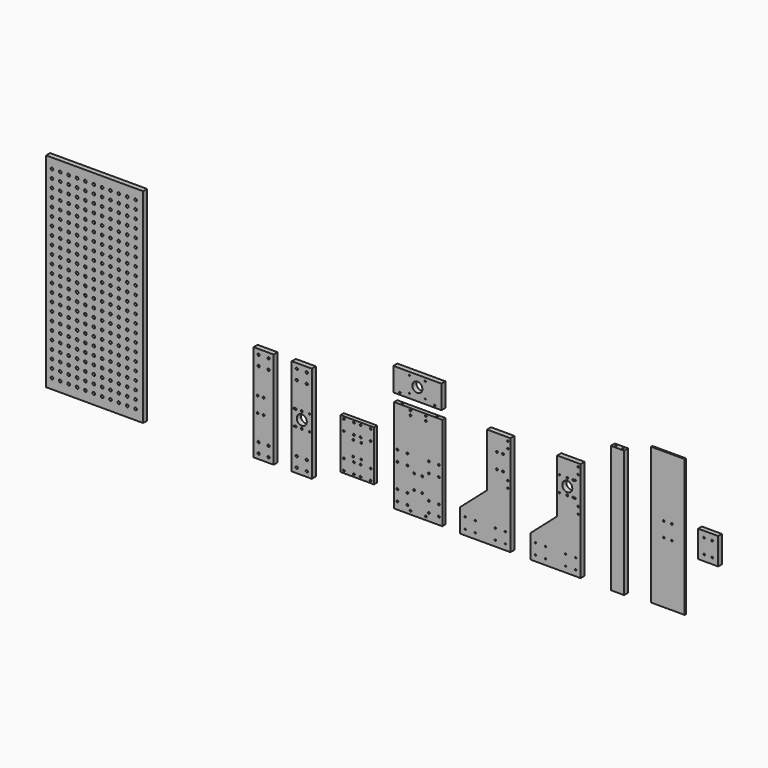
from build123d import *

# Parameters (mm, degrees)
F0_W     = 40
F0_H     = 380
F1_DEPTH = 15
F0_R     = 2.1
F0_R_2   = 2.25
F0_R_3   = 2
F0_R_4   = 2.75
F0_R_5   = 15
F0_W_2   = 60
F0_H_2   = 290
F0_R_6   = 3.4
F0_W_3   = 144
F0_H_3   = 70
F0_R_7   = 2.5
F0_R_8   = 1.8209797518
F0_R_9   = 1.6005552441
F0_R_10  = 1.752522135
F0_R_11  = 1.8797549558
F0_W_4   = 290
F0_H_4   = 610
F0_R_12  = 4
F0_W_5   = 100
F0_H_5   = 410
F2_DEPTH = 5
F0_H_6   = 280
F3_DEPTH = 12
F0_H_7   = 150
F0_H_8   = 80
F4_DEPTH = 14
F5_R     = 2.25
F6_DEPTH = 394.7827727966
F7_R     = 2.5
F8_DEPTH = 10


# Not quite as in the source:
# - a feature names something its author has since deleted; it is built from what else it names


with BuildPart() as f1:
    # F0 (on Front) → F1 (new body)
    with BuildSketch(Plane.XZ):
        with Locations((180, 65.6040832443)):
            Rectangle(F0_W, F0_H)
    extrude(amount=F1_DEPTH)

    # F5 (on face) → F6 (cut, through all)
    with BuildSketch(Plane.XY.offset(255.6040832443)):
        with Locations((170, -7.5)):
            Circle(F5_R)
        with Locations((190, -7.5)):
            Circle(F5_R)
    extrude(amount=-F6_DEPTH, mode=Mode.SUBTRACT)


with BuildPart() as f1b:
    # F0 (on Front) → F1, piece 2 (new body)
    with BuildSketch(Plane.XZ):
        Polygon((-80, -52), (-80, -122), (70, -122), (70, 178), (0, 178), (0, 18), align=None)
        with Locations((-65, -105)):
            Circle(F0_R, mode=Mode.SUBTRACT)
        with Locations((-35, -105)):
            Circle(F0_R, mode=Mode.SUBTRACT)
        with Locations((-65, -73)):
            Circle(F0_R, mode=Mode.SUBTRACT)
        with Locations((-35, -73)):
            Circle(F0_R, mode=Mode.SUBTRACT)
        with Locations((25, -105)):
            Circle(F0_R, mode=Mode.SUBTRACT)
        with Locations((55, -105)):
            Circle(F0_R, mode=Mode.SUBTRACT)
        with Locations((25, -73)):
            Circle(F0_R, mode=Mode.SUBTRACT)
        with Locations((55, -73)):
            Circle(F0_R, mode=Mode.SUBTRACT)
        with Locations((62.5, 44)):
            Circle(F0_R_2, mode=Mode.SUBTRACT)
        with Locations((62.5, 64)):
            Circle(F0_R_2, mode=Mode.SUBTRACT)
        with Locations((6.5, 82.5)):
            Circle(F0_R_3, mode=Mode.SUBTRACT)
        with Locations((30, 83)):
            Circle(F0_R_4, mode=Mode.SUBTRACT)
        with Locations((48, 83)):
            Circle(F0_R_4, mode=Mode.SUBTRACT)
        with Locations((53.5, 82.5)):
            Circle(F0_R_3, mode=Mode.SUBTRACT)
        with Locations((30, 106)):
            Circle(F0_R_5, mode=Mode.SUBTRACT)
        with Locations((6.5, 129.5)):
            Circle(F0_R_3, mode=Mode.SUBTRACT)
        with Locations((30, 129)):
            Circle(F0_R_4, mode=Mode.SUBTRACT)
        with Locations((48, 129)):
            Circle(F0_R_4, mode=Mode.SUBTRACT)
        with Locations((53.5, 130.2057206631)):
            Circle(F0_R_3, mode=Mode.SUBTRACT)
        with Locations((62.5, 148)):
            Circle(F0_R_2, mode=Mode.SUBTRACT)
        with Locations((62.5, 168)):
            Circle(F0_R_2, mode=Mode.SUBTRACT)
    extrude(amount=F1_DEPTH)


with BuildPart() as f1c:
    # F0 (on Front) → F1, piece 3 (new body)
    with BuildSketch(Plane.XZ):
        Polygon((-290, -52), (-290, -122), (-140, -122), (-140, 178), (-210, 178), (-210, 18), align=None)
        with Locations((-275, -105)):
            Circle(F0_R, mode=Mode.SUBTRACT)
        with Locations((-275, -73)):
            Circle(F0_R, mode=Mode.SUBTRACT)
        with Locations((-245, -105)):
            Circle(F0_R, mode=Mode.SUBTRACT)
        with Locations((-185, -105)):
            Circle(F0_R, mode=Mode.SUBTRACT)
        with Locations((-155, -105)):
            Circle(F0_R, mode=Mode.SUBTRACT)
        with Locations((-245, -73)):
            Circle(F0_R, mode=Mode.SUBTRACT)
        with Locations((-185, -73)):
            Circle(F0_R, mode=Mode.SUBTRACT)
        with Locations((-155, -73)):
            Circle(F0_R, mode=Mode.SUBTRACT)
        with Locations((-147.5, 44)):
            Circle(F0_R_2, mode=Mode.SUBTRACT)
        with Locations((-147.5, 64)):
            Circle(F0_R_2, mode=Mode.SUBTRACT)
        with Locations((-180, 83)):
            Circle(F0_R_4, mode=Mode.SUBTRACT)
        with Locations((-162, 83)):
            Circle(F0_R_4, mode=Mode.SUBTRACT)
        with Locations((-180, 129)):
            Circle(F0_R_4, mode=Mode.SUBTRACT)
        with Locations((-162, 129)):
            Circle(F0_R_4, mode=Mode.SUBTRACT)
        with Locations((-147.5, 148)):
            Circle(F0_R_2, mode=Mode.SUBTRACT)
        with Locations((-147.5, 168)):
            Circle(F0_R_2, mode=Mode.SUBTRACT)
    extrude(amount=F1_DEPTH)


with BuildPart() as f1d:
    # F0 (on Front) → F1, piece 4 (new body)
    with BuildSketch(Plane.XZ):
        with Locations((-763.4110760689, 23)):
            Rectangle(F0_W_2, F0_H_2)
        with Locations((-778.4110760689, -107)):
            Circle(F0_R_6, mode=Mode.SUBTRACT)
        with Locations((-778.4110760689, -77)):
            Circle(F0_R_6, mode=Mode.SUBTRACT)
        with Locations((-748.4110760689, -107)):
            Circle(F0_R_6, mode=Mode.SUBTRACT)
        with Locations((-748.4110760689, -77)):
            Circle(F0_R_6, mode=Mode.SUBTRACT)
        with Locations((-786.9110760689, -0.5)):
            Circle(F0_R_3, mode=Mode.SUBTRACT)
        with Locations((-781.4110760689, 0)):
            Circle(F0_R_4, mode=Mode.SUBTRACT)
        with Locations((-763.4110760689, 0)):
            Circle(F0_R_4, mode=Mode.SUBTRACT)
        with Locations((-739.9110760689, -0.5)):
            Circle(F0_R_3, mode=Mode.SUBTRACT)
        with Locations((-786.9110760689, 46.5)):
            Circle(F0_R_3, mode=Mode.SUBTRACT)
        with Locations((-781.4110760689, 46)):
            Circle(F0_R_4, mode=Mode.SUBTRACT)
        with Locations((-763.4110760689, 23)):
            Circle(F0_R_5, mode=Mode.SUBTRACT)
        with Locations((-763.4110760689, 46)):
            Circle(F0_R_4, mode=Mode.SUBTRACT)
        with Locations((-739.9110760689, 46.5)):
            Circle(F0_R_3, mode=Mode.SUBTRACT)
        with Locations((-778.4110760689, 123)):
            Circle(F0_R_6, mode=Mode.SUBTRACT)
        with Locations((-778.4110760689, 153)):
            Circle(F0_R_6, mode=Mode.SUBTRACT)
        with Locations((-748.4110760689, 123)):
            Circle(F0_R_6, mode=Mode.SUBTRACT)
        with Locations((-748.4110760689, 153)):
            Circle(F0_R_6, mode=Mode.SUBTRACT)
    extrude(amount=F1_DEPTH)


with BuildPart() as f1e:
    # F0 (on Front) → F1, piece 5 (new body)
    with BuildSketch(Plane.XZ):
        with Locations((-877.410800457, 23)):
            Rectangle(F0_W_2, F0_H_2)
        with Locations((-892.410800457, -107)):
            Circle(F0_R_6, mode=Mode.SUBTRACT)
        with Locations((-862.410800457, -107)):
            Circle(F0_R_6, mode=Mode.SUBTRACT)
        with Locations((-892.410800457, -77)):
            Circle(F0_R_6, mode=Mode.SUBTRACT)
        with Locations((-862.410800457, -77)):
            Circle(F0_R_6, mode=Mode.SUBTRACT)
        with Locations((-895.410800457, -1.2824487388)):
            Circle(F0_R_4, mode=Mode.SUBTRACT)
        with Locations((-877.410800457, -1.2824487388)):
            Circle(F0_R_4, mode=Mode.SUBTRACT)
        with Locations((-895.410800457, 44.7175512612)):
            Circle(F0_R_4, mode=Mode.SUBTRACT)
        with Locations((-877.410800457, 44.7175512612)):
            Circle(F0_R_4, mode=Mode.SUBTRACT)
        with Locations((-892.410800457, 123)):
            Circle(F0_R_6, mode=Mode.SUBTRACT)
        with Locations((-862.410800457, 123)):
            Circle(F0_R_6, mode=Mode.SUBTRACT)
        with Locations((-892.410800457, 153)):
            Circle(F0_R_6, mode=Mode.SUBTRACT)
        with Locations((-862.410800457, 153)):
            Circle(F0_R_6, mode=Mode.SUBTRACT)
    extrude(amount=F1_DEPTH)


with BuildPart() as f1f:
    # F0 (on Front) → F1, piece 6 (new body)
    with BuildSketch(Plane.XZ):
        with Locations((-418, 219.5401751995)):
            Rectangle(F0_W_3, F0_H_3)
        with Locations((-470, 190.5401751995)):
            Circle(F0_R_7, mode=Mode.SUBTRACT)
        with Locations((-441.5, 198.0401751995)):
            Circle(F0_R_8, mode=Mode.SUBTRACT)
        with Locations((-366, 190.5401751995)):
            Circle(F0_R_7, mode=Mode.SUBTRACT)
        with Locations((-394.5, 198.0401751995)):
            Circle(F0_R_9, mode=Mode.SUBTRACT)
        with Locations((-418, 221.5401751995)):
            Circle(F0_R_5, mode=Mode.SUBTRACT)
        with Locations((-441.5, 245.0401751995)):
            Circle(F0_R_10, mode=Mode.SUBTRACT)
        with Locations((-394.5, 245.0401751995)):
            Circle(F0_R_11, mode=Mode.SUBTRACT)
    extrude(amount=F1_DEPTH)


with BuildPart() as f1g:
    # F0 (on Front) → F1, piece 7 (new body)
    with BuildSketch(Plane.XZ):
        with Locations((-1382.5847482681, 165.8223104477)):
            Rectangle(F0_W_4, F0_H_4)
        with Locations((-1510.0847482681, -109.1776895523)):
            Circle(F0_R_12, mode=Mode.SUBTRACT)
        with Locations((-1485.0847482681, -109.1776895523)):
            Circle(F0_R_12, mode=Mode.SUBTRACT)
        with Locations((-1460.0847482681, -109.1776895523)):
            Circle(F0_R_12, mode=Mode.SUBTRACT)
        with Locations((-1435.0847482681, -109.1776895523)):
            Circle(F0_R_12, mode=Mode.SUBTRACT)
        with Locations((-1410.0847482681, -109.1776895523)):
            Circle(F0_R_12, mode=Mode.SUBTRACT)
        with Locations((-1385.0847482681, -109.1776895523)):
            Circle(F0_R_12, mode=Mode.SUBTRACT)
        with Locations((-1360.0847482681, -109.1776895523)):
            Circle(F0_R_12, mode=Mode.SUBTRACT)
        with Locations((-1335.0847482681, -109.1776895523)):
            Circle(F0_R_12, mode=Mode.SUBTRACT)
        with Locations((-1310.0847482681, -109.1776895523)):
            Circle(F0_R_12, mode=Mode.SUBTRACT)
        with Locations((-1285.0847482681, -109.1776895523)):
            Circle(F0_R_12, mode=Mode.SUBTRACT)
        with Locations((-1510.0847482681, -84.1776895523)):
            Circle(F0_R_12, mode=Mode.SUBTRACT)
        with Locations((-1485.0847482681, -84.1776895523)):
            Circle(F0_R_12, mode=Mode.SUBTRACT)
        with Locations((-1460.0847482681, -84.1776895523)):
            Circle(F0_R_12, mode=Mode.SUBTRACT)
        with Locations((-1435.0847482681, -84.1776895523)):
            Circle(F0_R_12, mode=Mode.SUBTRACT)
        with Locations((-1410.0847482681, -84.1776895523)):
            Circle(F0_R_12, mode=Mode.SUBTRACT)
        with Locations((-1385.0847482681, -84.1776895523)):
            Circle(F0_R_12, mode=Mode.SUBTRACT)
        with Locations((-1360.0847482681, -84.1776895523)):
            Circle(F0_R_12, mode=Mode.SUBTRACT)
        with Locations((-1335.0847482681, -84.1776895523)):
            Circle(F0_R_12, mode=Mode.SUBTRACT)
        with Locations((-1310.0847482681, -84.1776895523)):
            Circle(F0_R_12, mode=Mode.SUBTRACT)
        with Locations((-1285.0847482681, -84.1776895523)):
            Circle(F0_R_12, mode=Mode.SUBTRACT)
        with Locations((-1260.0847482681, -109.1776895523)):
            Circle(F0_R_12, mode=Mode.SUBTRACT)
        with Locations((-1260.0847482681, -84.1776895523)):
            Circle(F0_R_12, mode=Mode.SUBTRACT)
        with Locations((-1510.0847482681, -59.1776895523)):
            Circle(F0_R_12, mode=Mode.SUBTRACT)
        with Locations((-1485.0847482681, -59.1776895523)):
            Circle(F0_R_12, mode=Mode.SUBTRACT)
        with Locations((-1460.0847482681, -59.1776895523)):
            Circle(F0_R_12, mode=Mode.SUBTRACT)
        with Locations((-1435.0847482681, -59.1776895523)):
            Circle(F0_R_12, mode=Mode.SUBTRACT)
        with Locations((-1410.0847482681, -59.1776895523)):
            Circle(F0_R_12, mode=Mode.SUBTRACT)
        with Locations((-1510.0847482681, -34.1776895523)):
            Circle(F0_R_12, mode=Mode.SUBTRACT)
        with Locations((-1485.0847482681, -34.1776895523)):
            Circle(F0_R_12, mode=Mode.SUBTRACT)
        with Locations((-1460.0847482681, -34.1776895523)):
            Circle(F0_R_12, mode=Mode.SUBTRACT)
        with Locations((-1435.0847482681, -34.1776895523)):
            Circle(F0_R_12, mode=Mode.SUBTRACT)
        with Locations((-1410.0847482681, -34.1776895523)):
            Circle(F0_R_12, mode=Mode.SUBTRACT)
        with Locations((-1385.0847482681, -59.1776895523)):
            Circle(F0_R_12, mode=Mode.SUBTRACT)
        with Locations((-1360.0847482681, -59.1776895523)):
            Circle(F0_R_12, mode=Mode.SUBTRACT)
        with Locations((-1335.0847482681, -59.1776895523)):
            Circle(F0_R_12, mode=Mode.SUBTRACT)
        with Locations((-1310.0847482681, -59.1776895523)):
            Circle(F0_R_12, mode=Mode.SUBTRACT)
        with Locations((-1285.0847482681, -59.1776895523)):
            Circle(F0_R_12, mode=Mode.SUBTRACT)
        with Locations((-1385.0847482681, -34.1776895523)):
            Circle(F0_R_12, mode=Mode.SUBTRACT)
        with Locations((-1360.0847482681, -34.1776895523)):
            Circle(F0_R_12, mode=Mode.SUBTRACT)
        with Locations((-1335.0847482681, -34.1776895523)):
            Circle(F0_R_12, mode=Mode.SUBTRACT)
        with Locations((-1310.0847482681, -34.1776895523)):
            Circle(F0_R_12, mode=Mode.SUBTRACT)
        with Locations((-1285.0847482681, -34.1776895523)):
            Circle(F0_R_12, mode=Mode.SUBTRACT)
        with Locations((-1510.0847482681, -9.1776895523)):
            Circle(F0_R_12, mode=Mode.SUBTRACT)
        with Locations((-1485.0847482681, -9.1776895523)):
            Circle(F0_R_12, mode=Mode.SUBTRACT)
        with Locations((-1460.0847482681, -9.1776895523)):
            Circle(F0_R_12, mode=Mode.SUBTRACT)
        with Locations((-1435.0847482681, -9.1776895523)):
            Circle(F0_R_12, mode=Mode.SUBTRACT)
        with Locations((-1410.0847482681, -9.1776895523)):
            Circle(F0_R_12, mode=Mode.SUBTRACT)
        with Locations((-1385.0847482681, -9.1776895523)):
            Circle(F0_R_12, mode=Mode.SUBTRACT)
        with Locations((-1360.0847482681, -9.1776895523)):
            Circle(F0_R_12, mode=Mode.SUBTRACT)
        with Locations((-1335.0847482681, -9.1776895523)):
            Circle(F0_R_12, mode=Mode.SUBTRACT)
        with Locations((-1310.0847482681, -9.1776895523)):
            Circle(F0_R_12, mode=Mode.SUBTRACT)
        with Locations((-1285.0847482681, -9.1776895523)):
            Circle(F0_R_12, mode=Mode.SUBTRACT)
        with Locations((-1260.0847482681, -59.1776895523)):
            Circle(F0_R_12, mode=Mode.SUBTRACT)
        with Locations((-1260.0847482681, -34.1776895523)):
            Circle(F0_R_12, mode=Mode.SUBTRACT)
        with Locations((-1260.0847482681, -9.1776895523)):
            Circle(F0_R_12, mode=Mode.SUBTRACT)
        with Locations((-1510.0847482681, 15.8223104477)):
            Circle(F0_R_12, mode=Mode.SUBTRACT)
        with Locations((-1485.0847482681, 15.8223104477)):
            Circle(F0_R_12, mode=Mode.SUBTRACT)
        with Locations((-1460.0847482681, 15.8223104477)):
            Circle(F0_R_12, mode=Mode.SUBTRACT)
        with Locations((-1435.0847482681, 15.8223104477)):
            Circle(F0_R_12, mode=Mode.SUBTRACT)
        with Locations((-1410.0847482681, 15.8223104477)):
            Circle(F0_R_12, mode=Mode.SUBTRACT)
        with Locations((-1510.0847482681, 40.8223104477)):
            Circle(F0_R_12, mode=Mode.SUBTRACT)
        with Locations((-1485.0847482681, 40.8223104477)):
            Circle(F0_R_12, mode=Mode.SUBTRACT)
        with Locations((-1460.0847482681, 40.8223104477)):
            Circle(F0_R_12, mode=Mode.SUBTRACT)
        with Locations((-1435.0847482681, 40.8223104477)):
            Circle(F0_R_12, mode=Mode.SUBTRACT)
        with Locations((-1410.0847482681, 40.8223104477)):
            Circle(F0_R_12, mode=Mode.SUBTRACT)
        with Locations((-1385.0847482681, 15.8223104477)):
            Circle(F0_R_12, mode=Mode.SUBTRACT)
        with Locations((-1360.0847482681, 15.8223104477)):
            Circle(F0_R_12, mode=Mode.SUBTRACT)
        with Locations((-1335.0847482681, 15.8223104477)):
            Circle(F0_R_12, mode=Mode.SUBTRACT)
        with Locations((-1310.0847482681, 15.8223104477)):
            Circle(F0_R_12, mode=Mode.SUBTRACT)
        with Locations((-1285.0847482681, 15.8223104477)):
            Circle(F0_R_12, mode=Mode.SUBTRACT)
        with Locations((-1385.0847482681, 40.8223104477)):
            Circle(F0_R_12, mode=Mode.SUBTRACT)
        with Locations((-1360.0847482681, 40.8223104477)):
            Circle(F0_R_12, mode=Mode.SUBTRACT)
        with Locations((-1335.0847482681, 40.8223104477)):
            Circle(F0_R_12, mode=Mode.SUBTRACT)
        with Locations((-1310.0847482681, 40.8223104477)):
            Circle(F0_R_12, mode=Mode.SUBTRACT)
        with Locations((-1285.0847482681, 40.8223104477)):
            Circle(F0_R_12, mode=Mode.SUBTRACT)
        with Locations((-1510.0847482681, 65.8223104477)):
            Circle(F0_R_12, mode=Mode.SUBTRACT)
        with Locations((-1485.0847482681, 65.8223104477)):
            Circle(F0_R_12, mode=Mode.SUBTRACT)
        with Locations((-1460.0847482681, 65.8223104477)):
            Circle(F0_R_12, mode=Mode.SUBTRACT)
        with Locations((-1435.0847482681, 65.8223104477)):
            Circle(F0_R_12, mode=Mode.SUBTRACT)
        with Locations((-1410.0847482681, 65.8223104477)):
            Circle(F0_R_12, mode=Mode.SUBTRACT)
        with Locations((-1385.0847482681, 65.8223104477)):
            Circle(F0_R_12, mode=Mode.SUBTRACT)
        with Locations((-1360.0847482681, 65.8223104477)):
            Circle(F0_R_12, mode=Mode.SUBTRACT)
        with Locations((-1335.0847482681, 65.8223104477)):
            Circle(F0_R_12, mode=Mode.SUBTRACT)
        with Locations((-1310.0847482681, 65.8223104477)):
            Circle(F0_R_12, mode=Mode.SUBTRACT)
        with Locations((-1285.0847482681, 65.8223104477)):
            Circle(F0_R_12, mode=Mode.SUBTRACT)
        with Locations((-1260.0847482681, 15.8223104477)):
            Circle(F0_R_12, mode=Mode.SUBTRACT)
        with Locations((-1260.0847482681, 40.8223104477)):
            Circle(F0_R_12, mode=Mode.SUBTRACT)
        with Locations((-1260.0847482681, 65.8223104477)):
            Circle(F0_R_12, mode=Mode.SUBTRACT)
        with Locations((-1510.0847482681, 90.8223104477)):
            Circle(F0_R_12, mode=Mode.SUBTRACT)
        with Locations((-1485.0847482681, 90.8223104477)):
            Circle(F0_R_12, mode=Mode.SUBTRACT)
        with Locations((-1460.0847482681, 90.8223104477)):
            Circle(F0_R_12, mode=Mode.SUBTRACT)
        with Locations((-1435.0847482681, 90.8223104477)):
            Circle(F0_R_12, mode=Mode.SUBTRACT)
        with Locations((-1410.0847482681, 90.8223104477)):
            Circle(F0_R_12, mode=Mode.SUBTRACT)
        with Locations((-1510.0847482681, 115.8223104477)):
            Circle(F0_R_12, mode=Mode.SUBTRACT)
        with Locations((-1485.0847482681, 115.8223104477)):
            Circle(F0_R_12, mode=Mode.SUBTRACT)
        with Locations((-1460.0847482681, 115.8223104477)):
            Circle(F0_R_12, mode=Mode.SUBTRACT)
        with Locations((-1435.0847482681, 115.8223104477)):
            Circle(F0_R_12, mode=Mode.SUBTRACT)
        with Locations((-1410.0847482681, 115.8223104477)):
            Circle(F0_R_12, mode=Mode.SUBTRACT)
        with Locations((-1385.0847482681, 90.8223104477)):
            Circle(F0_R_12, mode=Mode.SUBTRACT)
        with Locations((-1360.0847482681, 90.8223104477)):
            Circle(F0_R_12, mode=Mode.SUBTRACT)
        with Locations((-1335.0847482681, 90.8223104477)):
            Circle(F0_R_12, mode=Mode.SUBTRACT)
        with Locations((-1310.0847482681, 90.8223104477)):
            Circle(F0_R_12, mode=Mode.SUBTRACT)
        with Locations((-1285.0847482681, 90.8223104477)):
            Circle(F0_R_12, mode=Mode.SUBTRACT)
        with Locations((-1385.0847482681, 115.8223104477)):
            Circle(F0_R_12, mode=Mode.SUBTRACT)
        with Locations((-1360.0847482681, 115.8223104477)):
            Circle(F0_R_12, mode=Mode.SUBTRACT)
        with Locations((-1335.0847482681, 115.8223104477)):
            Circle(F0_R_12, mode=Mode.SUBTRACT)
        with Locations((-1310.0847482681, 115.8223104477)):
            Circle(F0_R_12, mode=Mode.SUBTRACT)
        with Locations((-1285.0847482681, 115.8223104477)):
            Circle(F0_R_12, mode=Mode.SUBTRACT)
        with Locations((-1510.0847482681, 140.8223104477)):
            Circle(F0_R_12, mode=Mode.SUBTRACT)
        with Locations((-1485.0847482681, 140.8223104477)):
            Circle(F0_R_12, mode=Mode.SUBTRACT)
        with Locations((-1460.0847482681, 140.8223104477)):
            Circle(F0_R_12, mode=Mode.SUBTRACT)
        with Locations((-1435.0847482681, 140.8223104477)):
            Circle(F0_R_12, mode=Mode.SUBTRACT)
        with Locations((-1410.0847482681, 140.8223104477)):
            Circle(F0_R_12, mode=Mode.SUBTRACT)
        with Locations((-1385.0847482681, 140.8223104477)):
            Circle(F0_R_12, mode=Mode.SUBTRACT)
        with Locations((-1360.0847482681, 140.8223104477)):
            Circle(F0_R_12, mode=Mode.SUBTRACT)
        with Locations((-1335.0847482681, 140.8223104477)):
            Circle(F0_R_12, mode=Mode.SUBTRACT)
        with Locations((-1310.0847482681, 140.8223104477)):
            Circle(F0_R_12, mode=Mode.SUBTRACT)
        with Locations((-1285.0847482681, 140.8223104477)):
            Circle(F0_R_12, mode=Mode.SUBTRACT)
        with Locations((-1260.0847482681, 90.8223104477)):
            Circle(F0_R_12, mode=Mode.SUBTRACT)
        with Locations((-1260.0847482681, 115.8223104477)):
            Circle(F0_R_12, mode=Mode.SUBTRACT)
        with Locations((-1260.0847482681, 140.8223104477)):
            Circle(F0_R_12, mode=Mode.SUBTRACT)
        with Locations((-1510.0847482681, 165.8223104477)):
            Circle(F0_R_12, mode=Mode.SUBTRACT)
        with Locations((-1485.0847482681, 165.8223104477)):
            Circle(F0_R_12, mode=Mode.SUBTRACT)
        with Locations((-1460.0847482681, 165.8223104477)):
            Circle(F0_R_12, mode=Mode.SUBTRACT)
        with Locations((-1435.0847482681, 165.8223104477)):
            Circle(F0_R_12, mode=Mode.SUBTRACT)
        with Locations((-1410.0847482681, 165.8223104477)):
            Circle(F0_R_12, mode=Mode.SUBTRACT)
        with Locations((-1510.0847482681, 190.8223104477)):
            Circle(F0_R_12, mode=Mode.SUBTRACT)
        with Locations((-1485.0847482681, 190.8223104477)):
            Circle(F0_R_12, mode=Mode.SUBTRACT)
        with Locations((-1460.0847482681, 190.8223104477)):
            Circle(F0_R_12, mode=Mode.SUBTRACT)
        with Locations((-1435.0847482681, 190.8223104477)):
            Circle(F0_R_12, mode=Mode.SUBTRACT)
        with Locations((-1410.0847482681, 190.8223104477)):
            Circle(F0_R_12, mode=Mode.SUBTRACT)
        with Locations((-1385.0847482681, 165.8223104477)):
            Circle(F0_R_12, mode=Mode.SUBTRACT)
        with Locations((-1360.0847482681, 165.8223104477)):
            Circle(F0_R_12, mode=Mode.SUBTRACT)
        with Locations((-1335.0847482681, 165.8223104477)):
            Circle(F0_R_12, mode=Mode.SUBTRACT)
        with Locations((-1310.0847482681, 165.8223104477)):
            Circle(F0_R_12, mode=Mode.SUBTRACT)
        with Locations((-1285.0847482681, 165.8223104477)):
            Circle(F0_R_12, mode=Mode.SUBTRACT)
        with Locations((-1385.0847482681, 190.8223104477)):
            Circle(F0_R_12, mode=Mode.SUBTRACT)
        with Locations((-1360.0847482681, 190.8223104477)):
            Circle(F0_R_12, mode=Mode.SUBTRACT)
        with Locations((-1335.0847482681, 190.8223104477)):
            Circle(F0_R_12, mode=Mode.SUBTRACT)
        with Locations((-1310.0847482681, 190.8223104477)):
            Circle(F0_R_12, mode=Mode.SUBTRACT)
        with Locations((-1285.0847482681, 190.8223104477)):
            Circle(F0_R_12, mode=Mode.SUBTRACT)
        with Locations((-1510.0847482681, 215.8223104477)):
            Circle(F0_R_12, mode=Mode.SUBTRACT)
        with Locations((-1485.0847482681, 215.8223104477)):
            Circle(F0_R_12, mode=Mode.SUBTRACT)
        with Locations((-1460.0847482681, 215.8223104477)):
            Circle(F0_R_12, mode=Mode.SUBTRACT)
        with Locations((-1435.0847482681, 215.8223104477)):
            Circle(F0_R_12, mode=Mode.SUBTRACT)
        with Locations((-1410.0847482681, 215.8223104477)):
            Circle(F0_R_12, mode=Mode.SUBTRACT)
        with Locations((-1510.0847482681, 240.8223104477)):
            Circle(F0_R_12, mode=Mode.SUBTRACT)
        with Locations((-1485.0847482681, 240.8223104477)):
            Circle(F0_R_12, mode=Mode.SUBTRACT)
        with Locations((-1460.0847482681, 240.8223104477)):
            Circle(F0_R_12, mode=Mode.SUBTRACT)
        with Locations((-1435.0847482681, 240.8223104477)):
            Circle(F0_R_12, mode=Mode.SUBTRACT)
        with Locations((-1410.0847482681, 240.8223104477)):
            Circle(F0_R_12, mode=Mode.SUBTRACT)
        with Locations((-1385.0847482681, 215.8223104477)):
            Circle(F0_R_12, mode=Mode.SUBTRACT)
        with Locations((-1360.0847482681, 215.8223104477)):
            Circle(F0_R_12, mode=Mode.SUBTRACT)
        with Locations((-1335.0847482681, 215.8223104477)):
            Circle(F0_R_12, mode=Mode.SUBTRACT)
        with Locations((-1310.0847482681, 215.8223104477)):
            Circle(F0_R_12, mode=Mode.SUBTRACT)
        with Locations((-1285.0847482681, 215.8223104477)):
            Circle(F0_R_12, mode=Mode.SUBTRACT)
        with Locations((-1385.0847482681, 240.8223104477)):
            Circle(F0_R_12, mode=Mode.SUBTRACT)
        with Locations((-1360.0847482681, 240.8223104477)):
            Circle(F0_R_12, mode=Mode.SUBTRACT)
        with Locations((-1335.0847482681, 240.8223104477)):
            Circle(F0_R_12, mode=Mode.SUBTRACT)
        with Locations((-1310.0847482681, 240.8223104477)):
            Circle(F0_R_12, mode=Mode.SUBTRACT)
        with Locations((-1285.0847482681, 240.8223104477)):
            Circle(F0_R_12, mode=Mode.SUBTRACT)
        with Locations((-1260.0847482681, 165.8223104477)):
            Circle(F0_R_12, mode=Mode.SUBTRACT)
        with Locations((-1260.0847482681, 190.8223104477)):
            Circle(F0_R_12, mode=Mode.SUBTRACT)
        with Locations((-1260.0847482681, 215.8223104477)):
            Circle(F0_R_12, mode=Mode.SUBTRACT)
        with Locations((-1260.0847482681, 240.8223104477)):
            Circle(F0_R_12, mode=Mode.SUBTRACT)
        with Locations((-1510.0847482681, 265.8223104477)):
            Circle(F0_R_12, mode=Mode.SUBTRACT)
        with Locations((-1485.0847482681, 265.8223104477)):
            Circle(F0_R_12, mode=Mode.SUBTRACT)
        with Locations((-1460.0847482681, 265.8223104477)):
            Circle(F0_R_12, mode=Mode.SUBTRACT)
        with Locations((-1435.0847482681, 265.8223104477)):
            Circle(F0_R_12, mode=Mode.SUBTRACT)
        with Locations((-1410.0847482681, 265.8223104477)):
            Circle(F0_R_12, mode=Mode.SUBTRACT)
        with Locations((-1385.0847482681, 265.8223104477)):
            Circle(F0_R_12, mode=Mode.SUBTRACT)
        with Locations((-1360.0847482681, 265.8223104477)):
            Circle(F0_R_12, mode=Mode.SUBTRACT)
        with Locations((-1335.0847482681, 265.8223104477)):
            Circle(F0_R_12, mode=Mode.SUBTRACT)
        with Locations((-1310.0847482681, 265.8223104477)):
            Circle(F0_R_12, mode=Mode.SUBTRACT)
        with Locations((-1285.0847482681, 265.8223104477)):
            Circle(F0_R_12, mode=Mode.SUBTRACT)
        with Locations((-1510.0847482681, 290.8223104477)):
            Circle(F0_R_12, mode=Mode.SUBTRACT)
        with Locations((-1485.0847482681, 290.8223104477)):
            Circle(F0_R_12, mode=Mode.SUBTRACT)
        with Locations((-1460.0847482681, 290.8223104477)):
            Circle(F0_R_12, mode=Mode.SUBTRACT)
        with Locations((-1435.0847482681, 290.8223104477)):
            Circle(F0_R_12, mode=Mode.SUBTRACT)
        with Locations((-1410.0847482681, 290.8223104477)):
            Circle(F0_R_12, mode=Mode.SUBTRACT)
        with Locations((-1510.0847482681, 315.8223104477)):
            Circle(F0_R_12, mode=Mode.SUBTRACT)
        with Locations((-1485.0847482681, 315.8223104477)):
            Circle(F0_R_12, mode=Mode.SUBTRACT)
        with Locations((-1460.0847482681, 315.8223104477)):
            Circle(F0_R_12, mode=Mode.SUBTRACT)
        with Locations((-1435.0847482681, 315.8223104477)):
            Circle(F0_R_12, mode=Mode.SUBTRACT)
        with Locations((-1410.0847482681, 315.8223104477)):
            Circle(F0_R_12, mode=Mode.SUBTRACT)
        with Locations((-1385.0847482681, 290.8223104477)):
            Circle(F0_R_12, mode=Mode.SUBTRACT)
        with Locations((-1360.0847482681, 290.8223104477)):
            Circle(F0_R_12, mode=Mode.SUBTRACT)
        with Locations((-1335.0847482681, 290.8223104477)):
            Circle(F0_R_12, mode=Mode.SUBTRACT)
        with Locations((-1310.0847482681, 290.8223104477)):
            Circle(F0_R_12, mode=Mode.SUBTRACT)
        with Locations((-1285.0847482681, 290.8223104477)):
            Circle(F0_R_12, mode=Mode.SUBTRACT)
        with Locations((-1385.0847482681, 315.8223104477)):
            Circle(F0_R_12, mode=Mode.SUBTRACT)
        with Locations((-1360.0847482681, 315.8223104477)):
            Circle(F0_R_12, mode=Mode.SUBTRACT)
        with Locations((-1335.0847482681, 315.8223104477)):
            Circle(F0_R_12, mode=Mode.SUBTRACT)
        with Locations((-1310.0847482681, 315.8223104477)):
            Circle(F0_R_12, mode=Mode.SUBTRACT)
        with Locations((-1285.0847482681, 315.8223104477)):
            Circle(F0_R_12, mode=Mode.SUBTRACT)
        with Locations((-1260.0847482681, 265.8223104477)):
            Circle(F0_R_12, mode=Mode.SUBTRACT)
        with Locations((-1260.0847482681, 290.8223104477)):
            Circle(F0_R_12, mode=Mode.SUBTRACT)
        with Locations((-1260.0847482681, 315.8223104477)):
            Circle(F0_R_12, mode=Mode.SUBTRACT)
        with Locations((-1510.0847482681, 340.8223104477)):
            Circle(F0_R_12, mode=Mode.SUBTRACT)
        with Locations((-1485.0847482681, 340.8223104477)):
            Circle(F0_R_12, mode=Mode.SUBTRACT)
        with Locations((-1460.0847482681, 340.8223104477)):
            Circle(F0_R_12, mode=Mode.SUBTRACT)
        with Locations((-1435.0847482681, 340.8223104477)):
            Circle(F0_R_12, mode=Mode.SUBTRACT)
        with Locations((-1410.0847482681, 340.8223104477)):
            Circle(F0_R_12, mode=Mode.SUBTRACT)
        with Locations((-1385.0847482681, 340.8223104477)):
            Circle(F0_R_12, mode=Mode.SUBTRACT)
        with Locations((-1360.0847482681, 340.8223104477)):
            Circle(F0_R_12, mode=Mode.SUBTRACT)
        with Locations((-1335.0847482681, 340.8223104477)):
            Circle(F0_R_12, mode=Mode.SUBTRACT)
        with Locations((-1310.0847482681, 340.8223104477)):
            Circle(F0_R_12, mode=Mode.SUBTRACT)
        with Locations((-1285.0847482681, 340.8223104477)):
            Circle(F0_R_12, mode=Mode.SUBTRACT)
        with Locations((-1510.0847482681, 365.8223104477)):
            Circle(F0_R_12, mode=Mode.SUBTRACT)
        with Locations((-1485.0847482681, 365.8223104477)):
            Circle(F0_R_12, mode=Mode.SUBTRACT)
        with Locations((-1460.0847482681, 365.8223104477)):
            Circle(F0_R_12, mode=Mode.SUBTRACT)
        with Locations((-1435.0847482681, 365.8223104477)):
            Circle(F0_R_12, mode=Mode.SUBTRACT)
        with Locations((-1410.0847482681, 365.8223104477)):
            Circle(F0_R_12, mode=Mode.SUBTRACT)
        with Locations((-1510.0847482681, 390.8223104477)):
            Circle(F0_R_12, mode=Mode.SUBTRACT)
        with Locations((-1485.0847482681, 390.8223104477)):
            Circle(F0_R_12, mode=Mode.SUBTRACT)
        with Locations((-1460.0847482681, 390.8223104477)):
            Circle(F0_R_12, mode=Mode.SUBTRACT)
        with Locations((-1435.0847482681, 390.8223104477)):
            Circle(F0_R_12, mode=Mode.SUBTRACT)
        with Locations((-1410.0847482681, 390.8223104477)):
            Circle(F0_R_12, mode=Mode.SUBTRACT)
        with Locations((-1385.0847482681, 365.8223104477)):
            Circle(F0_R_12, mode=Mode.SUBTRACT)
        with Locations((-1360.0847482681, 365.8223104477)):
            Circle(F0_R_12, mode=Mode.SUBTRACT)
        with Locations((-1335.0847482681, 365.8223104477)):
            Circle(F0_R_12, mode=Mode.SUBTRACT)
        with Locations((-1310.0847482681, 365.8223104477)):
            Circle(F0_R_12, mode=Mode.SUBTRACT)
        with Locations((-1285.0847482681, 365.8223104477)):
            Circle(F0_R_12, mode=Mode.SUBTRACT)
        with Locations((-1385.0847482681, 390.8223104477)):
            Circle(F0_R_12, mode=Mode.SUBTRACT)
        with Locations((-1360.0847482681, 390.8223104477)):
            Circle(F0_R_12, mode=Mode.SUBTRACT)
        with Locations((-1335.0847482681, 390.8223104477)):
            Circle(F0_R_12, mode=Mode.SUBTRACT)
        with Locations((-1310.0847482681, 390.8223104477)):
            Circle(F0_R_12, mode=Mode.SUBTRACT)
        with Locations((-1285.0847482681, 390.8223104477)):
            Circle(F0_R_12, mode=Mode.SUBTRACT)
        with Locations((-1260.0847482681, 340.8223104477)):
            Circle(F0_R_12, mode=Mode.SUBTRACT)
        with Locations((-1260.0847482681, 365.8223104477)):
            Circle(F0_R_12, mode=Mode.SUBTRACT)
        with Locations((-1260.0847482681, 390.8223104477)):
            Circle(F0_R_12, mode=Mode.SUBTRACT)
        with Locations((-1510.0847482681, 415.8223104477)):
            Circle(F0_R_12, mode=Mode.SUBTRACT)
        with Locations((-1485.0847482681, 415.8223104477)):
            Circle(F0_R_12, mode=Mode.SUBTRACT)
        with Locations((-1460.0847482681, 415.8223104477)):
            Circle(F0_R_12, mode=Mode.SUBTRACT)
        with Locations((-1435.0847482681, 415.8223104477)):
            Circle(F0_R_12, mode=Mode.SUBTRACT)
        with Locations((-1410.0847482681, 415.8223104477)):
            Circle(F0_R_12, mode=Mode.SUBTRACT)
        with Locations((-1385.0847482681, 415.8223104477)):
            Circle(F0_R_12, mode=Mode.SUBTRACT)
        with Locations((-1360.0847482681, 415.8223104477)):
            Circle(F0_R_12, mode=Mode.SUBTRACT)
        with Locations((-1335.0847482681, 415.8223104477)):
            Circle(F0_R_12, mode=Mode.SUBTRACT)
        with Locations((-1310.0847482681, 415.8223104477)):
            Circle(F0_R_12, mode=Mode.SUBTRACT)
        with Locations((-1285.0847482681, 415.8223104477)):
            Circle(F0_R_12, mode=Mode.SUBTRACT)
        with Locations((-1510.0847482681, 440.8223104477)):
            Circle(F0_R_12, mode=Mode.SUBTRACT)
        with Locations((-1485.0847482681, 440.8223104477)):
            Circle(F0_R_12, mode=Mode.SUBTRACT)
        with Locations((-1460.0847482681, 440.8223104477)):
            Circle(F0_R_12, mode=Mode.SUBTRACT)
        with Locations((-1435.0847482681, 440.8223104477)):
            Circle(F0_R_12, mode=Mode.SUBTRACT)
        with Locations((-1410.0847482681, 440.8223104477)):
            Circle(F0_R_12, mode=Mode.SUBTRACT)
        with Locations((-1385.0847482681, 440.8223104477)):
            Circle(F0_R_12, mode=Mode.SUBTRACT)
        with Locations((-1360.0847482681, 440.8223104477)):
            Circle(F0_R_12, mode=Mode.SUBTRACT)
        with Locations((-1335.0847482681, 440.8223104477)):
            Circle(F0_R_12, mode=Mode.SUBTRACT)
        with Locations((-1310.0847482681, 440.8223104477)):
            Circle(F0_R_12, mode=Mode.SUBTRACT)
        with Locations((-1285.0847482681, 440.8223104477)):
            Circle(F0_R_12, mode=Mode.SUBTRACT)
        with Locations((-1260.0847482681, 415.8223104477)):
            Circle(F0_R_12, mode=Mode.SUBTRACT)
        with Locations((-1260.0847482681, 440.8223104477)):
            Circle(F0_R_12, mode=Mode.SUBTRACT)
    extrude(amount=F1_DEPTH)


with BuildPart() as f2:
    # F0 (on Front) → F2 (new body)
    with BuildSketch(Plane.XZ):
        with Locations((322.7434039116, 80.6040832443)):
            Rectangle(F0_W_5, F0_H_5)
        with Locations((310.7434039116, 58.6040832443)):
            Circle(F0_R_7, mode=Mode.SUBTRACT)
        with Locations((334.7434039116, 58.6040832443)):
            Circle(F0_R_7, mode=Mode.SUBTRACT)
        with Locations((310.7434039116, 102.6040832443)):
            Circle(F0_R_7, mode=Mode.SUBTRACT)
        with Locations((334.7434039116, 102.6040832443)):
            Circle(F0_R_7, mode=Mode.SUBTRACT)
    extrude(amount=F2_DEPTH)


with BuildPart() as f3:
    # F0 (on Front) → F3 (new body)
    with BuildSketch(Plane.XZ):
        with Locations((-418, 18)):
            Rectangle(F0_W_3, F0_H_6)
        with Locations((-441, -112)):
            Circle(F0_R_4, mode=Mode.SUBTRACT)
        with Locations((-395, -112)):
            Circle(F0_R_4, mode=Mode.SUBTRACT)
        with Locations((-480, -100)):
            Circle(F0_R_4, mode=Mode.SUBTRACT)
        with Locations((-450, -100)):
            Circle(F0_R_4, mode=Mode.SUBTRACT)
        with Locations((-480, -68)):
            Circle(F0_R_4, mode=Mode.SUBTRACT)
        with Locations((-450, -68)):
            Circle(F0_R_4, mode=Mode.SUBTRACT)
        with Locations((-386, -100)):
            Circle(F0_R_4, mode=Mode.SUBTRACT)
        with Locations((-356, -100)):
            Circle(F0_R_4, mode=Mode.SUBTRACT)
        with Locations((-386, -68)):
            Circle(F0_R_4, mode=Mode.SUBTRACT)
        with Locations((-356, -68)):
            Circle(F0_R_4, mode=Mode.SUBTRACT)
        with Locations((-430, -54)):
            Circle(F0_R_4, mode=Mode.SUBTRACT)
        with Locations((-406, -54)):
            Circle(F0_R_4, mode=Mode.SUBTRACT)
        with Locations((-430, -10)):
            Circle(F0_R_4, mode=Mode.SUBTRACT)
        with Locations((-406, -10)):
            Circle(F0_R_4, mode=Mode.SUBTRACT)
        with Locations((-480, 4)):
            Circle(F0_R_4, mode=Mode.SUBTRACT)
        with Locations((-450, 4)):
            Circle(F0_R_4, mode=Mode.SUBTRACT)
        with Locations((-386, 4)):
            Circle(F0_R_4, mode=Mode.SUBTRACT)
        with Locations((-356, 4)):
            Circle(F0_R_4, mode=Mode.SUBTRACT)
        with Locations((-480, 36)):
            Circle(F0_R_4, mode=Mode.SUBTRACT)
        with Locations((-450, 36)):
            Circle(F0_R_4, mode=Mode.SUBTRACT)
        with Locations((-386, 36)):
            Circle(F0_R_4, mode=Mode.SUBTRACT)
        with Locations((-356, 36)):
            Circle(F0_R_4, mode=Mode.SUBTRACT)
        with Locations((-441, 139)):
            Circle(F0_R_4, mode=Mode.SUBTRACT)
        with Locations((-441, 152)):
            Circle(F0_R_4, mode=Mode.SUBTRACT)
        with Locations((-395, 139)):
            Circle(F0_R_4, mode=Mode.SUBTRACT)
        with Locations((-395, 152)):
            Circle(F0_R_4, mode=Mode.SUBTRACT)
    extrude(amount=F3_DEPTH)

    # F7 (on face) → F8 (cut)
    with BuildSketch(Plane.XY.offset(158)):
        with Locations((-470, -6)):
            Circle(F7_R)
        with Locations((-366, -6)):
            Circle(F7_R)
    extrude(amount=-F8_DEPTH, mode=Mode.SUBTRACT)


with BuildPart() as f3b:
    # F0 (on Front) → F3, piece 2 (new body)
    with BuildSketch(Plane.XZ):
        with Locations((-600, -3.1741780639)):
            Rectangle(F0_W_5, F0_H_7)
        with Locations((-640, -71.1741780639)):
            Circle(F0_R_4, mode=Mode.SUBTRACT)
        with Locations((-610, -71.1741780639)):
            Circle(F0_R_4, mode=Mode.SUBTRACT)
        with Locations((-590, -71.1741780639)):
            Circle(F0_R_4, mode=Mode.SUBTRACT)
        with Locations((-560, -71.1741780639)):
            Circle(F0_R_4, mode=Mode.SUBTRACT)
        with Locations((-640, -39.1741780639)):
            Circle(F0_R_4, mode=Mode.SUBTRACT)
        with Locations((-610, -39.1741780639)):
            Circle(F0_R_4, mode=Mode.SUBTRACT)
        with Locations((-590, -39.1741780639)):
            Circle(F0_R_4, mode=Mode.SUBTRACT)
        with Locations((-612, -25.1741780639)):
            Circle(F0_R_4, mode=Mode.SUBTRACT)
        with Locations((-588, -25.1741780639)):
            Circle(F0_R_4, mode=Mode.SUBTRACT)
        with Locations((-560, -39.1741780639)):
            Circle(F0_R_4, mode=Mode.SUBTRACT)
        with Locations((-612, 18.8258219361)):
            Circle(F0_R_4, mode=Mode.SUBTRACT)
        with Locations((-588, 18.8258219361)):
            Circle(F0_R_4, mode=Mode.SUBTRACT)
        with Locations((-640, 32.8258219361)):
            Circle(F0_R_4, mode=Mode.SUBTRACT)
        with Locations((-610, 32.8258219361)):
            Circle(F0_R_4, mode=Mode.SUBTRACT)
        with Locations((-590, 32.8258219361)):
            Circle(F0_R_4, mode=Mode.SUBTRACT)
        with Locations((-560, 32.8258219361)):
            Circle(F0_R_4, mode=Mode.SUBTRACT)
        with Locations((-640, 64.8258219361)):
            Circle(F0_R_4, mode=Mode.SUBTRACT)
        with Locations((-610, 64.8258219361)):
            Circle(F0_R_4, mode=Mode.SUBTRACT)
        with Locations((-590, 64.8258219361)):
            Circle(F0_R_4, mode=Mode.SUBTRACT)
        with Locations((-560, 64.8258219361)):
            Circle(F0_R_4, mode=Mode.SUBTRACT)
    extrude(amount=F3_DEPTH)


with BuildPart() as f4:
    # F0 (on Front) → F4 (new body)
    with BuildSketch(Plane.XZ):
        with Locations((450.1988875866, 81.75)):
            Rectangle(F0_W_2, F0_H_8)
        with Locations((438.1988875866, 59.75)):
            Circle(F0_R_7, mode=Mode.SUBTRACT)
        with Locations((462.1988875866, 59.75)):
            Circle(F0_R_7, mode=Mode.SUBTRACT)
        with Locations((438.1988875866, 103.75)):
            Circle(F0_R_7, mode=Mode.SUBTRACT)
        with Locations((462.1988875866, 103.75)):
            Circle(F0_R_7, mode=Mode.SUBTRACT)
    extrude(amount=F4_DEPTH)


solid = Compound([f1.part, f1b.part, f1c.part, f1d.part, f1e.part, f1f.part, f1g.part, f2.part, f3.part, f3b.part, f4.part])
